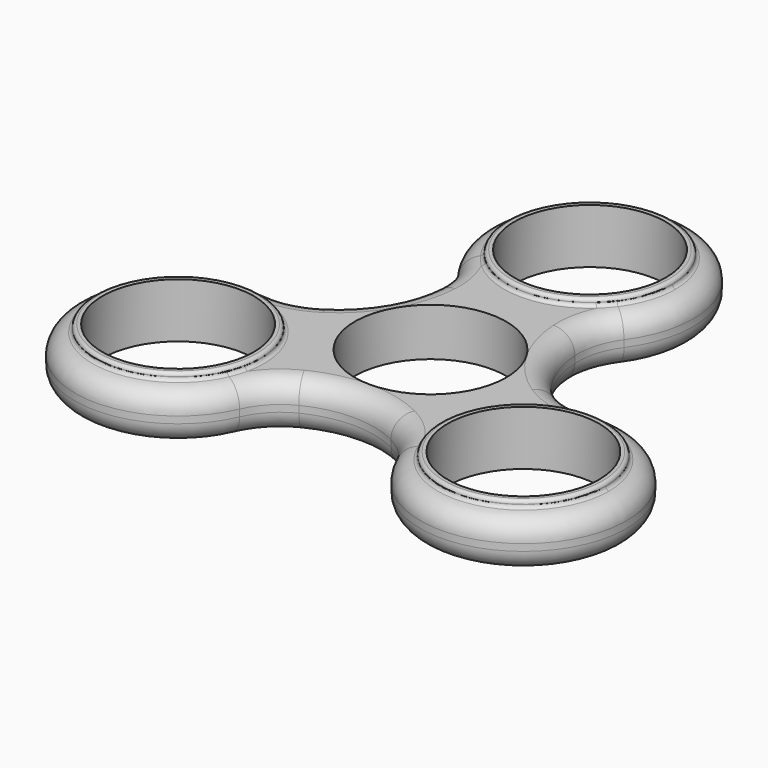
from build123d import *

# Parameters (mm, degrees)
F0_R         = 12.075
F0_R_2       = 11.075
F1_DEPTH     = 8
F2_DEPTH     = 7
F4_R         = 10
F5_T3_ANGLE  = 39.9143560654
F5_T6_ANGLE  = 39.9143560654
F5_T9_ANGLE  = 52.9990296168
F5_T12_ANGLE = 39.9143560654
F5_T15_ANGLE = 252.8277417874
F5_T18_ANGLE = 252.8277417874
F5_T21_ANGLE = 39.9143560654
F5_T24_ANGLE = 39.9143560654
F5_T27_ANGLE = 52.9990296168
F5_T30_ANGLE = 52.9990296168
F5_T33_ANGLE = 39.9143560654
F5_T36_ANGLE = 39.9143560654
F5_T39_ANGLE = 252.8277417874
F5_T42_ANGLE = 52.9990296168
F5_T45_ANGLE = 39.9143560654
F5_T48_ANGLE = 252.8277417874
F5_T51_ANGLE = 252.8277417874
F5_T54_ANGLE = 39.9143560654
F5_T57_ANGLE = 39.9143560654
F5_T60_ANGLE = 52.9990296168
F5_T63_ANGLE = 52.9990296168
F5_T66_ANGLE = 39.9143560654
F5_T69_ANGLE = 39.9143560654
F5_T72_ANGLE = 252.8277417874
F6_R         = 0.49999


# Not quite as in the source:
# - a fillet or chamfer that OpenCascade refuses, or shapes differently, is made with other operations: its cross-section is extruded or revolved along the edge and cut away or added
# - a fillet or chamfer is up to 0.001 mm smaller than in the source, because OpenCascade refuses the exact size


with BuildPart() as f1:
    # F0 (on Top) → F1 (new body)
    with BuildSketch(Plane.XY):
        with Locations((-80.4774807177, 29.15)):
            Circle(F0_R)
        with Locations((-80.4774807177, 29.15)):
            Circle(F0_R_2, mode=Mode.SUBTRACT)
    extrude(amount=F1_DEPTH)



with BuildPart() as f1b:
    # F0 (on Top) → F1, piece 2 (new body)
    with BuildSketch(Plane.XY):
        with Locations((-105.722121238, -14.575)):
            Circle(F0_R)
        with Locations((-105.722121238, -14.575)):
            Circle(F0_R_2, mode=Mode.SUBTRACT)
    extrude(amount=F1_DEPTH)


with BuildPart() as f1c:
    # F0 (on Top) → F1, piece 3 (new body)
    with BuildSketch(Plane.XY):
        with Locations((-55.2328401974, -14.575)):
            Circle(F0_R)
        with Locations((-55.2328401974, -14.575)):
            Circle(F0_R_2, mode=Mode.SUBTRACT)
    extrude(amount=F1_DEPTH)


with BuildPart() as f1_1:
    add(f1.part)

    add(f1b.part)  # F2 merges F1b

    add(f1c.part)  # F2 merges F1c
    # F0 (on Top) → F2 (join)
    with BuildSketch(Plane.XY):
        with BuildLine():
            ThreePointArc((-59.083164859, 0), (-68.2881731594, 7.0375), (-69.7803227883, 18.5280210302))
            ThreePointArc((-69.7803227883, 18.5280210302), (-80.4774807177, 44.225), (-91.174638647, 18.5280210302))
            ThreePointArc((-91.174638647, 18.5280210302), (-92.6667882759, 7.0375), (-101.8717965764, 0))
            ThreePointArc((-101.8717965764, 0), (-118.7774542, -22.1125), (-91.174638647, -18.5280210302))
            ThreePointArc((-91.174638647, -18.5280210302), (-80.4774807177, -14.075), (-69.7803227883, -18.5280210302))
            ThreePointArc((-69.7803227883, -18.5280210302), (-42.1775072353, -22.1125), (-59.083164859, 0))
        make_face()
        with Locations((-105.722121238, -14.575)):
            Circle(F0_R, mode=Mode.SUBTRACT)
        with Locations((-55.2328401974, -14.575)):
            Circle(F0_R, mode=Mode.SUBTRACT)
        with Locations((-80.4774807177, 0)):
            Circle(F0_R_2, mode=Mode.SUBTRACT)
        with Locations((-80.4774807177, 29.15)):
            Circle(F0_R, mode=Mode.SUBTRACT)
    extrude(amount=F2_DEPTH)

    # F3: union 

    # F4
    f4_edges = [f1_1.edges().sort_by_distance(p)[0] for p in [
        (-91.174639, -18.528021, 3.5),
        (-69.780323, -18.528021, 3.5),
        (-69.780323, 18.528021, 3.5),
        (-59.083165, 0, 3.5),
        (-91.174639, 18.528021, 3.5),
        (-101.871797, 0, 3.5),
    ]]
    fillet(f4_edges, radius=F4_R)

    # F5: fillet of radius 3 on 24 edges, made by hand


with BuildPart() as f5_tool1:
    # F5_s2 → F5_t3 (revolve)
    with BuildSketch(Plane(origin=(-1.0941509525, 17.8867242457, 0), x_dir=(0, 0, 1), z_dir=(0.0610569918, -0.9981342814, 0))):
        with BuildLine():
            ThreePointArc((7, 72.314885607), (6.1213203436, 70.1935652634), (4, 69.314885607))
            Line((4, 69.314885607), (7, 69.3148856067))
            Line((7, 69.3148856067), (7, 72.314885607))
        make_face()
    revolve(axis=Axis((-60.2983716707, 14.2651357645, 7), (0, 0, -1)), revolution_arc=F5_T3_ANGLE)


with BuildPart() as f5_tool4:
    # F5_s5 → F5_t6 (revolve)
    with BuildSketch(Plane(origin=(-1.0941509525, 17.8867242457, 0), x_dir=(0, 0, 1), z_dir=(0.0610569918, -0.9981342814, 0))):
        with BuildLine():
            ThreePointArc((3, 69.314885607), (0.8786796564, 70.1935652634), (0, 72.314885607))
            Line((0, 72.314885607), (0, 69.3148856067))
            Line((0, 69.3148856067), (3, 69.314885607))
        make_face()
    revolve(axis=Axis((-60.2983716707, 14.2651357645, 0), (0, 0, -1)), revolution_arc=F5_T6_ANGLE)


with BuildPart() as f5_tool7:
    # F5_s8 → F5_t9 (revolve)
    with BuildSketch(Plane(origin=(-45.1148118907, 29.8613919996, 0), x_dir=(0, 0, 1), z_dir=(0.8338811481, -0.5519440468, 0))):
        with BuildLine():
            ThreePointArc((7, 36.4066196006), (6.1213203436, 34.285299257), (4, 33.4066196006))
            Line((4, 33.4066196006), (7, 33.4066196006))
            Line((7, 33.4066196006), (7, 36.4066196006))
        make_face()
    revolve(axis=Axis((-55.2328401974, 14.575, 7), (0, 0, -1)), revolution_arc=F5_T9_ANGLE)


with BuildPart() as f5_tool10:
    # F5_s11 → F5_t12 (revolve)
    with BuildSketch(Plane(origin=(-45.1148119007, 29.861391995, 0), x_dir=(0, 0, 1), z_dir=(-0.8338811482, 0.5519440467, 0))):
        with BuildLine():
            ThreePointArc((7, -36.4066195915), (6.1213203436, -34.2852992479), (4, -33.4066195915))
            Line((4, -33.4066195915), (7, -33.4066195912))
            Line((7, -33.4066195912), (7, -36.4066195915))
        make_face()
    revolve(axis=Axis((-58.0339562337, 10.3430531782, 7), (0, 0, 1)), revolution_arc=F5_T12_ANGLE)


with BuildPart() as f5_tool13:
    # F5_s14 → F5_t15 (revolve)
    with BuildSketch(Plane(origin=(-3.4982164092, 8.0123877809, 0), x_dir=(0, 0, 1), z_dir=(-0.400127176, 0.9164596243, 0))):
        with BuildLine():
            ThreePointArc((7, -68.5255215677), (6.1213203436, -70.6468419113), (4, -71.5255215677))
            Line((4, -71.5255215677), (7, -71.5255215677))
            Line((7, -71.5255215677), (7, -68.5255215677))
        make_face()
    revolve(axis=Axis((-55.2328401974, -14.575, 7), (0, 0, 1)), revolution_arc=F5_T15_ANGLE)


with BuildPart() as f5_tool16:
    # F5_s17 → F5_t18 (revolve)
    with BuildSketch(Plane(origin=(-14.4331666999, -19.5667518414, 0), x_dir=(0, 0, 1), z_dir=(-0.5936137282, -0.8047501114, 0))):
        with BuildLine():
            ThreePointArc((7, 69.9931017452), (6.1213203436, 67.8717814016), (4, 66.9931017452))
            Line((4, 66.9931017452), (7, 66.9931017452))
            Line((7, 66.9931017452), (7, 69.9931017452))
        make_face()
    revolve(axis=Axis((-80.4774807177, 29.15, 7), (0, 0, 1)), revolution_arc=F5_T18_ANGLE)


with BuildPart() as f5_tool19:
    # F5_s20 → F5_t21 (revolve)
    with BuildSketch(Plane(origin=(-52.8155990726, 26.3323278975, 0), x_dir=(0, 0, 1), z_dir=(-0.89493814, 0.4461902348, 0))):
        with BuildLine():
            ThreePointArc((7, -43.9207127956), (6.1213203436, -46.0420331392), (4, -46.9207127956))
            Line((4, -46.9207127956), (7, -46.9207127959))
            Line((7, -46.9207127959), (7, -43.9207127956))
        make_face()
    revolve(axis=Axis((-78.2130652807, -24.6081889427, 7), (0, 0, -1)), revolution_arc=F5_T21_ANGLE)


with BuildPart() as f5_tool22:
    # F5_s23 → F5_t24 (revolve)
    with BuildSketch(Plane(origin=(-42.2837013009, 57.3231576822, 0), x_dir=(0, 0, 1), z_dir=(-0.593613728, 0.8047501115, 0))):
        with BuildLine():
            ThreePointArc((7, -59.5354214045), (6.1213203436, -61.6567417481), (4, -62.5354214045))
            Line((4, -62.5354214045), (7, -62.5354214048))
            Line((7, -62.5354214048), (7, -59.5354214045))
        make_face()
    revolve(axis=Axis((-100.6565897647, 14.2651357645, 7), (0, 0, -1)), revolution_arc=F5_T24_ANGLE)


with BuildPart() as f5_tool25:
    # F5_s26 → F5_t27 (revolve)
    with BuildSketch(Plane(origin=(-76.0955270856, -37.9390256868, 0), x_dir=(0, 0, 1), z_dir=(-0.8949381401, -0.4461902346, 0))):
        with BuildLine():
            ThreePointArc((7, 27.8958192203), (6.1213203436, 25.7744988767), (4, 24.8958192203))
            Line((4, 24.8958192203), (7, 24.8958192203))
            Line((7, 24.8958192203), (7, 27.8958192203))
        make_face()
    revolve(axis=Axis((-80.4774807177, -29.15, 7), (0, 0, -1)), revolution_arc=F5_T27_ANGLE)


with BuildPart() as f5_tool28:
    # F5_s29 → F5_t30 (revolve)
    with BuildSketch(Plane(origin=(0.4941178998, 8.0776336872, 0), x_dir=(0, 0, 1), z_dir=(0.0610569919, 0.9981342814, 0))):
        with BuildLine():
            ThreePointArc((7, -88.3397791689), (6.1213203436, -90.4610995125), (4, -91.3397791689))
            Line((4, -91.3397791689), (7, -91.3397791689))
            Line((7, -91.3397791689), (7, -88.3397791689))
        make_face()
    revolve(axis=Axis((-105.722121238, 14.575, 7), (0, 0, -1)), revolution_arc=F5_T30_ANGLE)


with BuildPart() as f5_tool31:
    # F5_s32 → F5_t33 (revolve)
    with BuildSketch(Plane(origin=(-22.2709557296, -51.009861198, 0), x_dir=(0, 0, 1), z_dir=(-0.4001271762, -0.9164596242, 0))):
        with BuildLine():
            ThreePointArc((7, 78.9832019111), (6.1213203436, 76.8618815675), (4, 75.9832019111))
            Line((4, 75.9832019111), (7, 75.9832019108))
            Line((7, 75.9832019108), (7, 78.9832019111))
        make_face()
    revolve(axis=Axis((-82.7418961547, -24.6081889427, 7), (0, 0, -1)), revolution_arc=F5_T33_ANGLE)


with BuildPart() as f5_tool34:
    # F5_s35 → F5_t36 (revolve)
    with BuildSketch(Plane(origin=(-66.8064710514, -44.2190521432, 0), x_dir=(0, 0, 1), z_dir=(0.8338811482, 0.5519440467, 0))):
        with BuildLine():
            ThreePointArc((7, -52.4315131518), (6.1213203436, -54.5528334953), (4, -55.4315131518))
            Line((4, -55.4315131518), (7, -55.4315131521))
            Line((7, -55.4315131521), (7, -52.4315131518))
        make_face()
    revolve(axis=Axis((-102.9210052017, 10.3430531782, 7), (0, 0, -1)), revolution_arc=F5_T36_ANGLE)


with BuildPart() as f5_tool37:
    # F5_s38 → F5_t39 (revolve)
    with BuildSketch(Plane(origin=(-102.7848379675, 11.5543640605, 0), x_dir=(0, 0, 1), z_dir=(0.9937409042, -0.111709513, 0))):
        with BuildLine():
            ThreePointArc((7, 14.2189403516), (6.1213203436, 12.0976200081), (4, 11.2189403516))
            Line((4, 11.2189403516), (7, 11.2189403516))
            Line((7, 11.2189403516), (7, 14.2189403516))
        make_face()
    revolve(axis=Axis((-105.722121238, -14.575, 7), (0, 0, 1)), revolution_arc=F5_T39_ANGLE)


with BuildPart() as f5_tool40:
    # F5_s41 → F5_t42 (revolve)
    with BuildSketch(Plane(origin=(-45.1148118907, 29.8613919996, 0), x_dir=(0, 0, 1), z_dir=(0.8338811481, -0.5519440468, 0))):
        with BuildLine():
            ThreePointArc((3, 33.4066196006), (0.8786796564, 34.285299257), (0, 36.4066196006))
            Line((0, 36.4066196006), (0, 33.4066196006))
            Line((0, 33.4066196006), (3, 33.4066196006))
        make_face()
    revolve(axis=Axis((-55.2328401974, 14.575, 0), (0, 0, -1)), revolution_arc=F5_T42_ANGLE)


with BuildPart() as f5_tool43:
    # F5_s44 → F5_t45 (revolve)
    with BuildSketch(Plane(origin=(-45.1148119007, 29.861391995, 0), x_dir=(0, 0, 1), z_dir=(-0.8338811482, 0.5519440467, 0))):
        with BuildLine():
            ThreePointArc((3, -33.4066195915), (0.8786796564, -34.2852992479), (0, -36.4066195915))
            Line((0, -36.4066195915), (0, -33.4066195912))
            Line((0, -33.4066195912), (3, -33.4066195915))
        make_face()
    revolve(axis=Axis((-58.0339562337, 10.3430531782, 0), (0, 0, 1)), revolution_arc=F5_T45_ANGLE)


with BuildPart() as f5_tool46:
    # F5_s47 → F5_t48 (revolve)
    with BuildSketch(Plane(origin=(-3.4982164092, 8.0123877809, 0), x_dir=(0, 0, 1), z_dir=(-0.400127176, 0.9164596243, 0))):
        with BuildLine():
            ThreePointArc((3, -71.5255215677), (0.8786796564, -70.6468419113), (0, -68.5255215677))
            Line((0, -68.5255215677), (0, -71.5255215677))
            Line((0, -71.5255215677), (3, -71.5255215677))
        make_face()
    revolve(axis=Axis((-55.2328401974, -14.575, 0), (0, 0, 1)), revolution_arc=F5_T48_ANGLE)


with BuildPart() as f5_tool49:
    # F5_s50 → F5_t51 (revolve)
    with BuildSketch(Plane(origin=(-14.4331666999, -19.5667518414, 0), x_dir=(0, 0, 1), z_dir=(-0.5936137282, -0.8047501114, 0))):
        with BuildLine():
            ThreePointArc((3, 66.9931017452), (0.8786796564, 67.8717814016), (0, 69.9931017452))
            Line((0, 69.9931017452), (0, 66.9931017452))
            Line((0, 66.9931017452), (3, 66.9931017452))
        make_face()
    revolve(axis=Axis((-80.4774807177, 29.15, 0), (0, 0, 1)), revolution_arc=F5_T51_ANGLE)


with BuildPart() as f5_tool52:
    # F5_s53 → F5_t54 (revolve)
    with BuildSketch(Plane(origin=(-52.8155990726, 26.3323278975, 0), x_dir=(0, 0, 1), z_dir=(-0.89493814, 0.4461902348, 0))):
        with BuildLine():
            ThreePointArc((3, -46.9207127956), (0.8786796564, -46.0420331392), (0, -43.9207127956))
            Line((0, -43.9207127956), (0, -46.9207127959))
            Line((0, -46.9207127959), (3, -46.9207127956))
        make_face()
    revolve(axis=Axis((-78.2130652807, -24.6081889427, 0), (0, 0, -1)), revolution_arc=F5_T54_ANGLE)


with BuildPart() as f5_tool55:
    # F5_s56 → F5_t57 (revolve)
    with BuildSketch(Plane(origin=(-42.2837013009, 57.3231576822, 0), x_dir=(0, 0, 1), z_dir=(-0.593613728, 0.8047501115, 0))):
        with BuildLine():
            ThreePointArc((3, -62.5354214045), (0.8786796564, -61.6567417481), (0, -59.5354214045))
            Line((0, -59.5354214045), (0, -62.5354214048))
            Line((0, -62.5354214048), (3, -62.5354214045))
        make_face()
    revolve(axis=Axis((-100.6565897647, 14.2651357645, 0), (0, 0, -1)), revolution_arc=F5_T57_ANGLE)


with BuildPart() as f5_tool58:
    # F5_s59 → F5_t60 (revolve)
    with BuildSketch(Plane(origin=(-76.0955270856, -37.9390256868, 0), x_dir=(0, 0, 1), z_dir=(-0.8949381401, -0.4461902346, 0))):
        with BuildLine():
            ThreePointArc((3, 24.8958192203), (0.8786796564, 25.7744988767), (0, 27.8958192203))
            Line((0, 27.8958192203), (0, 24.8958192203))
            Line((0, 24.8958192203), (3, 24.8958192203))
        make_face()
    revolve(axis=Axis((-80.4774807177, -29.15, 0), (0, 0, -1)), revolution_arc=F5_T60_ANGLE)


with BuildPart() as f5_tool61:
    # F5_s62 → F5_t63 (revolve)
    with BuildSketch(Plane(origin=(0.4941178998, 8.0776336872, 0), x_dir=(0, 0, 1), z_dir=(0.0610569919, 0.9981342814, 0))):
        with BuildLine():
            ThreePointArc((3, -91.3397791689), (0.8786796564, -90.4610995125), (0, -88.3397791689))
            Line((0, -88.3397791689), (0, -91.3397791689))
            Line((0, -91.3397791689), (3, -91.3397791689))
        make_face()
    revolve(axis=Axis((-105.722121238, 14.575, 0), (0, 0, -1)), revolution_arc=F5_T63_ANGLE)


with BuildPart() as f5_tool64:
    # F5_s65 → F5_t66 (revolve)
    with BuildSketch(Plane(origin=(-22.2709557296, -51.009861198, 0), x_dir=(0, 0, 1), z_dir=(-0.4001271762, -0.9164596242, 0))):
        with BuildLine():
            ThreePointArc((3, 75.9832019111), (0.8786796564, 76.8618815675), (0, 78.9832019111))
            Line((0, 78.9832019111), (0, 75.9832019108))
            Line((0, 75.9832019108), (3, 75.9832019111))
        make_face()
    revolve(axis=Axis((-82.7418961547, -24.6081889427, 0), (0, 0, -1)), revolution_arc=F5_T66_ANGLE)


with BuildPart() as f5_tool67:
    # F5_s68 → F5_t69 (revolve)
    with BuildSketch(Plane(origin=(-66.8064710514, -44.2190521432, 0), x_dir=(0, 0, 1), z_dir=(0.8338811482, 0.5519440467, 0))):
        with BuildLine():
            ThreePointArc((3, -55.4315131518), (0.8786796564, -54.5528334953), (0, -52.4315131518))
            Line((0, -52.4315131518), (0, -55.4315131521))
            Line((0, -55.4315131521), (3, -55.4315131518))
        make_face()
    revolve(axis=Axis((-102.9210052017, 10.3430531782, 0), (0, 0, -1)), revolution_arc=F5_T69_ANGLE)


with BuildPart() as f5_tool70:
    # F5_s71 → F5_t72 (revolve)
    with BuildSketch(Plane(origin=(-102.7848379675, 11.5543640605, 0), x_dir=(0, 0, 1), z_dir=(0.9937409042, -0.111709513, 0))):
        with BuildLine():
            ThreePointArc((3, 11.2189403516), (0.8786796564, 12.0976200081), (0, 14.2189403516))
            Line((0, 14.2189403516), (0, 11.2189403516))
            Line((0, 11.2189403516), (3, 11.2189403516))
        make_face()
    revolve(axis=Axis((-105.722121238, -14.575, 0), (0, 0, 1)), revolution_arc=F5_T72_ANGLE)


with BuildPart() as f1_2:
    add(f1_1.part)

    # F5_t73: cut F5_tool1, F5_tool4, F5_tool7, F5_tool10, F5_tool13, F5_tool16, F5_tool19, F5_tool22, F5_tool25, F5_tool28, F5_tool31, F5_tool34, F5_tool37, F5_tool40, F5_tool43, F5_tool46, F5_tool49, F5_tool52, F5_tool55, F5_tool58, F5_tool61, F5_tool64, F5_tool67, F5_tool70
    add([f5_tool1.part, f5_tool4.part, f5_tool7.part, f5_tool10.part, f5_tool13.part, f5_tool16.part, f5_tool19.part, f5_tool22.part, f5_tool25.part, f5_tool28.part, f5_tool31.part, f5_tool34.part, f5_tool37.part, f5_tool40.part, f5_tool43.part, f5_tool46.part, f5_tool49.part, f5_tool52.part, f5_tool55.part, f5_tool58.part, f5_tool61.part, f5_tool64.part, f5_tool67.part, f5_tool70.part], mode=Mode.SUBTRACT)

    # F6 (radius 0.5 in the source; OpenCascade refuses exactly that, so slightly less here)
    f6_edges = [f1_2.edges().sort_by_distance(p)[0] for p in [
        (-117.797121, -14.575, 8),
        (-92.552481, 29.15, 8),
        (-67.30784, -14.575, 8),
        (-52.764981, -26.395123, 7),
        (-47.18555, -5.572403, 7),
        (-69.007025, 25.377167, 7),
        (-84.250313, 40.620456, 7),
        (-65.690097, -8.5375, 7),
        (-68.402481, 29.15, 7.5),
        (-80.477481, 17.075, 7),
        (-116.179378, -20.6125, 7),
        (-96.719524, -6.52771, 7),
    ]]
    fillet(f6_edges, radius=F6_R)


solid = f1_2.part
